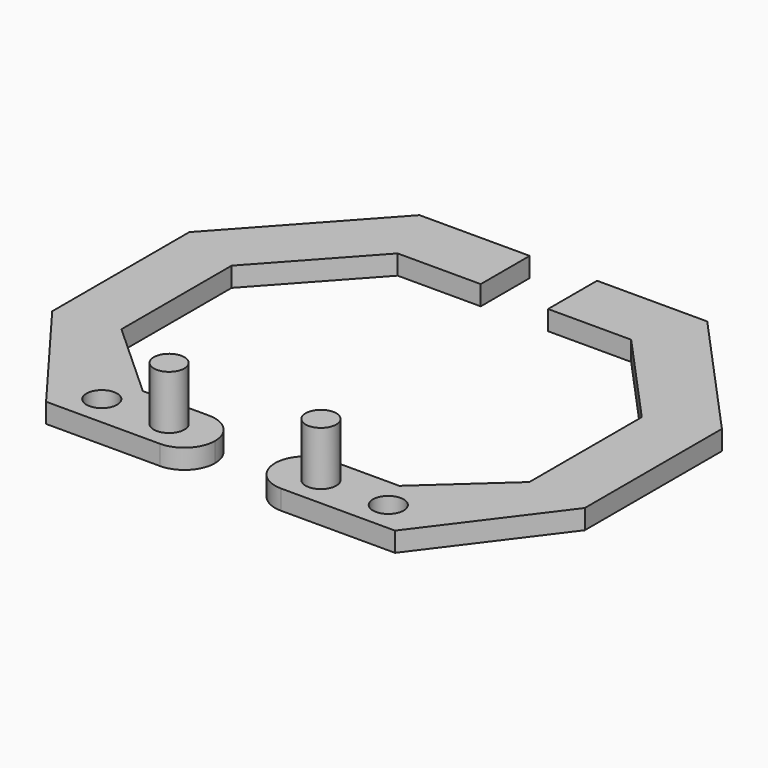
from build123d import *

# Parameters (mm, degrees)
F0_R     = 2.5
F1_DEPTH = 3.2
F2_DEPTH = 12
F3_DEPTH = 12
F4_R     = 4.99999
F5_R     = 4.99999


# Not quite as in the source:
# - a fillet or chamfer is up to 0.001 mm smaller than in the source, because OpenCascade refuses the exact size


with BuildPart() as f1:
    # F0 (on Top) → F1 (new body)
    with BuildSketch(Plane.XY):
        Polygon((4.9, -35), (28.5, -35), (43.5, -15), (43.5, 13), (23.5, 35), (5.5, 35), (5.5, 25), (19.0763011388, 25), (33.5, 9.1339312527), (33.5, -13.8162449002), (21.1978693902, -25), (4.9, -25), align=None)
        with Locations((12.4, -30)):
            Circle(F0_R, mode=Mode.SUBTRACT)
        with Locations((23.4, -30)):
            Circle(F0_R, mode=Mode.SUBTRACT)
    extrude(amount=F1_DEPTH)

    # F0 (on Top) → F2 (join)
    with BuildSketch(Plane.XY):
        with Locations((12.4, -30)):
            Circle(F0_R)
    extrude(amount=F2_DEPTH)

    # F4 (radius 5 in the source; OpenCascade refuses exactly that, so slightly less here)
    f4_edges = [f1.edges().sort_by_distance(p)[0] for p in [
        (4.9, -35, 1.6),
        (4.9, -25, 1.6),
    ]]
    fillet(f4_edges, radius=F4_R)


with BuildPart() as f1b:
    # F0 (on Top) → F1, piece 2 (new body)
    with BuildSketch(Plane.XY):
        Polygon((-28.5, -35), (-4.9, -35), (-4.9, -25), (-20.6968208253, -25), (-33.5, -13.3607462049), (-33.5, 9.1339312527), (-19.0763011388, 25), (-5.5, 25), (-5.5, 35), (-23.5, 35), (-43.5, 13), (-43.5, -15), align=None)
        with Locations((-23.4, -30)):
            Circle(F0_R, mode=Mode.SUBTRACT)
        with Locations((-12.4, -30)):
            Circle(F0_R, mode=Mode.SUBTRACT)
    extrude(amount=F1_DEPTH)

    # F0 (on Top) → F3 (join)
    with BuildSketch(Plane.XY):
        with Locations((-12.4, -30)):
            Circle(F0_R)
    extrude(amount=F3_DEPTH)

    # F5 (radius 5 in the source; OpenCascade refuses exactly that, so slightly less here)
    f5_edges = [f1b.edges().sort_by_distance(p)[0] for p in [
        (-4.9, -35, 1.6),
        (-4.9, -25, 1.6),
    ]]
    fillet(f5_edges, radius=F5_R)


solid = Compound([f1.part, f1b.part])
